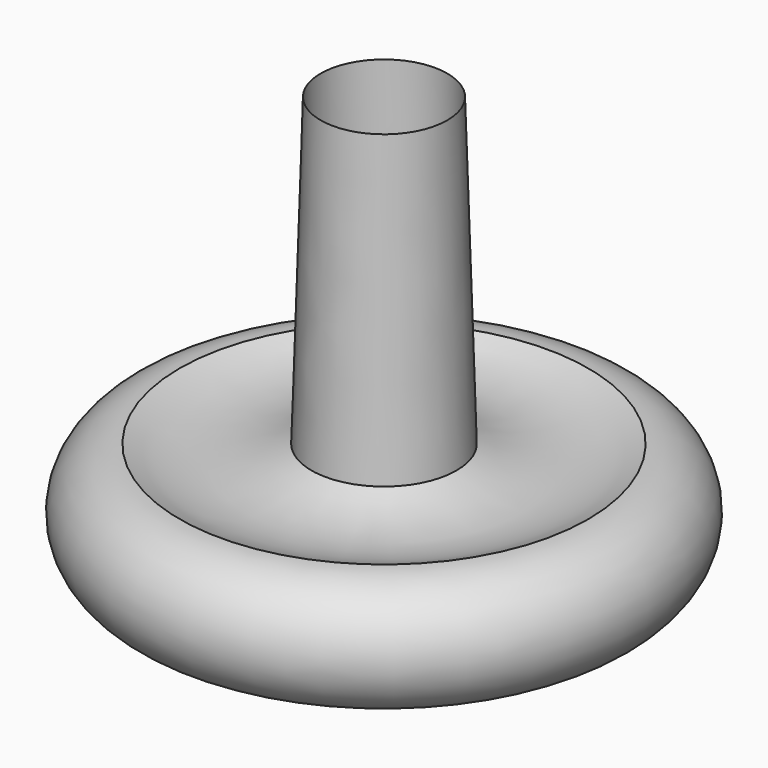
from build123d import *

# Parameters (mm, degrees)
F2_R      = 4.7625
F1_FACE_R = 7.62
F3_DEPTH  = 9.525
F4_DEPTH  = 22.225


# Not quite as in the source:
# - a feature names something its author has since deleted; it is built from what else it names


with BuildPart() as f1:
    # F0 (on Front) → F1 (revolve)
    with BuildSketch(Plane.XZ):
        with BuildLine():
            Line((0, 58.42), (0, 0))
            Line((0, 0), (9.8843732849, 7.3464941233))
            Line((9.8843732849, 7.3464941233), (24.5773624629, 7.3464941233))
            ThreePointArc((24.5773624629, 7.3464941233), (31.75, 14.5191316605), (24.5773624629, 21.6917691976))
            ThreePointArc((24.5773624629, 21.6917691976), (16.6510342816, 19.7936922223), (8.7247061003, 21.6917691976))
            Line((8.7247061003, 21.6917691976), (7.62, 58.42))
            Line((7.62, 58.42), (0, 58.42))
        make_face()
    revolve(axis=Axis((0, 0, 29.21), (0, 0, -1)))

    # F2 (on Top) + F1_face (on face) → F3 (cut)
    with BuildSketch(Plane.XY):
        Circle(F2_R)
    with BuildSketch(Plane.XY.offset(58.42)):
        Circle(F1_FACE_R)
    extrude(amount=-F3_DEPTH, mode=Mode.SUBTRACT)

    # F2 (on Top) → F4 (cut)
    with BuildSketch(Plane.XY):
        Circle(F2_R)
    extrude(amount=F4_DEPTH, mode=Mode.SUBTRACT)


solid = f1.part
